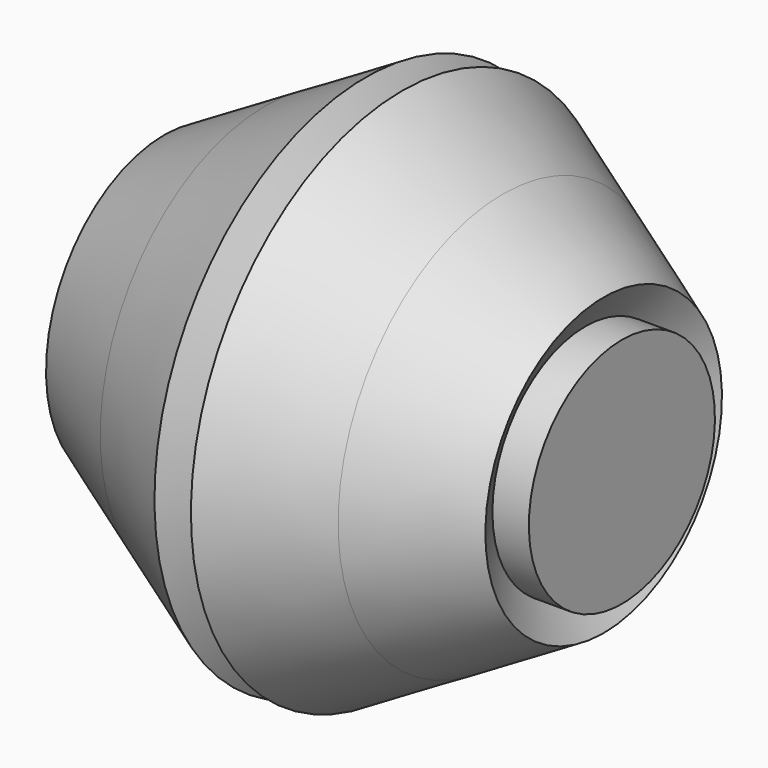
from build123d import *

# Parameters (mm, degrees)
F0_W = 80
F0_H = 80


# Not quite as in the source:
# - after a boolean that leaves OpenCascade's solid faulty, fix() repairs it


with BuildPart() as f1:
    # F0 (on Front) → F1 (revolve)
    with BuildSketch(Plane.XZ):
        with Locations((207.3035305738, 40)):
            Rectangle(F0_W, F0_H)
        Polygon((194.7596802331, -32.4445538099), (125.4776479304, -72.4445538099), (165.4776479304, -141.7265861126), (234.7596802331, -101.7265861126), align=None)
        with Locations((-40, -40)):
            Rectangle(F0_W, F0_H)
        Polygon((111.1079149462, -112.4445538099), (41.8258826435, -72.4445538099), (1.8258826435, -141.7265861126), (71.1079149462, -181.7265861126), align=None)
        Polygon((125.4776479304, 72.4445538099), (165.4776479304, 141.7265861126), (96.1956156276, 181.7265861126), (56.1956156276, 112.4445538099), align=None)
        Polygon((41.8258826435, 72.4445538099), (1.8258826435, 141.7265861126), (-67.4561496593, 101.7265861126), (-27.4561496593, 32.4445538099), align=None)
    revolve(axis=Axis((207.3035305738, 0, 0), (-1, 0, 0)))

    add(f1.part.fix(), mode=Mode.REPLACE)


solid = f1.part
